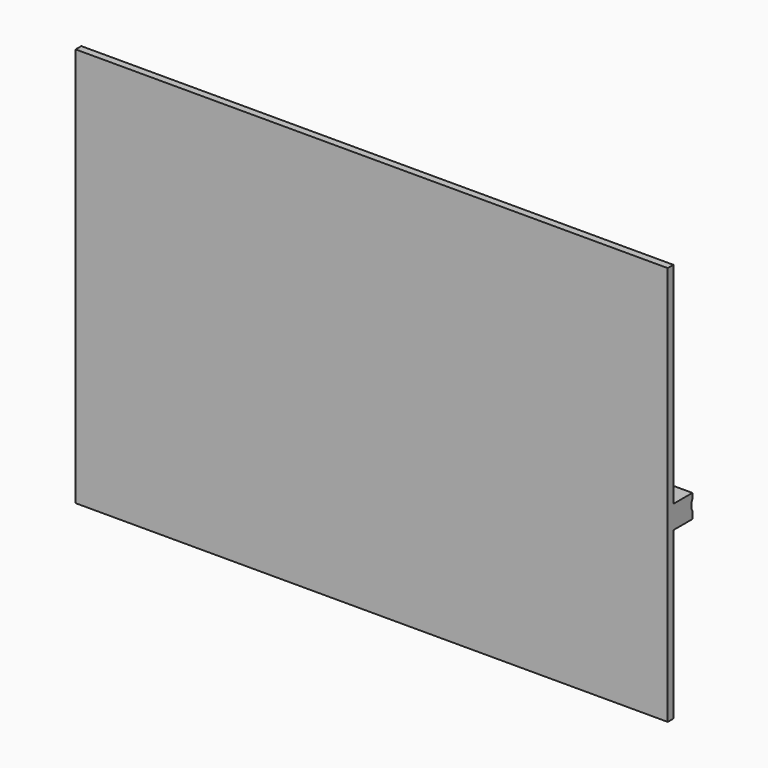
from build123d import *

# Parameters (mm, degrees)
F0_W     = 83
F0_H     = 56
F1_DEPTH = 1
F3_DEPTH = 83


# Not quite as in the source:
# - a feature names something its author has since deleted; it is built from what else it names


with BuildPart() as f1:
    # F0 (on Front) → F1 (new body)
    with BuildSketch(Plane.XZ):
        Rectangle(F0_W, F0_H)
    extrude(amount=F1_DEPTH)

    # F2 (on face) → F3 (join)
    with BuildSketch(Plane.YZ.offset(41.5)):
        with BuildLine():
            ThreePointArc((3.3219824545, -3.733111607), (3.130625787, -3), (3.3219824545, -2.266888393))
            Line((3.3219824545, -2.266888393), (3.3219824545, -1.492598909))
            Line((3.3219824545, -1.492598909), (0, -1.492598909))
            Line((0, -1.492598909), (0, -4.7320667654))
            Line((0, -4.7320667654), (3.3219824545, -4.7320667654))
            Line((3.3219824545, -4.7320667654), (3.3219824545, -3.733111607))
        make_face()
        with BuildLine():
            ThreePointArc((0, 27.0385164807), (-0.1, 26.5), (0, 25.9614835193))
            Line((0, 25.9614835193), (0, 27.0385164807))
        make_face()
    extrude(amount=-F3_DEPTH)


solid = f1.part
